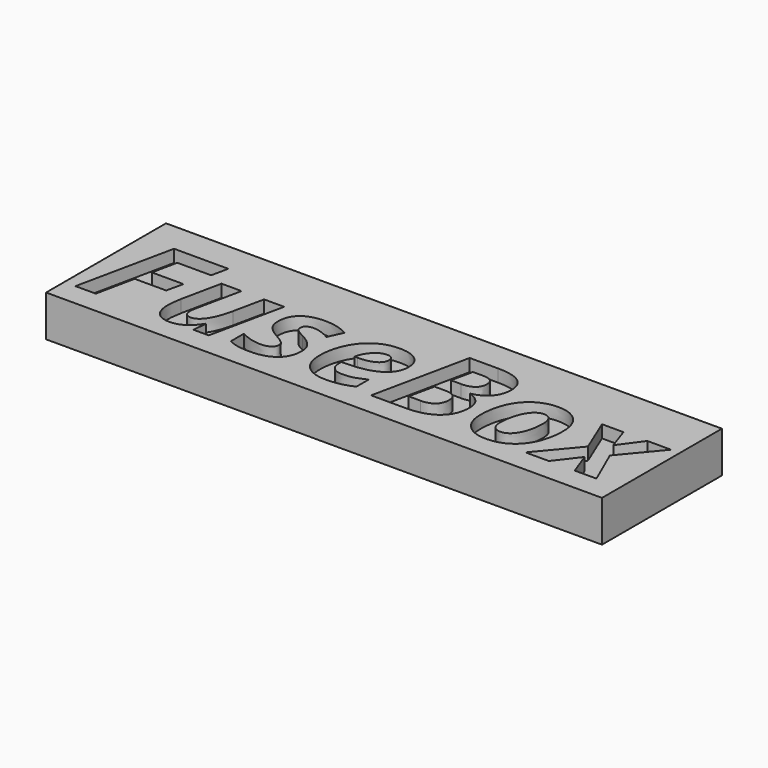
from build123d import *

# Parameters (mm, degrees)
F0_W         = 44.5
F0_H         = 12
F1_DEPTH     = 3.3
F2_TEXT_SIZE = 10.9305106715
F3_DEPTH     = 1


# Not quite as in the source:
# - Text() gives the source's letters only with a copy of the font that has no kerning and outlines rounded to 1/6400 em; it was checked with that copy


with BuildPart() as f1:
    # F0 (on Top) → F1 (new body)
    with BuildSketch(Plane.XY):
        with Locations((11.3993290961, 0.1862416454)):
            Rectangle(F0_W, F0_H)
    extrude(amount=F1_DEPTH)

    # F2 (on face) → F3 (cut)
    with BuildSketch(Plane.XY.offset(3.3)):
        with Locations((-10.2400870346, -3.9936397225)):
            Text('FuseBox', F2_TEXT_SIZE, font='Open Sans', font_style=FontStyle.BOLDITALIC, text_align=(TextAlign.LEFT, TextAlign.BOTTOM))
    extrude(amount=-F3_DEPTH, mode=Mode.SUBTRACT)


solid = f1.part
